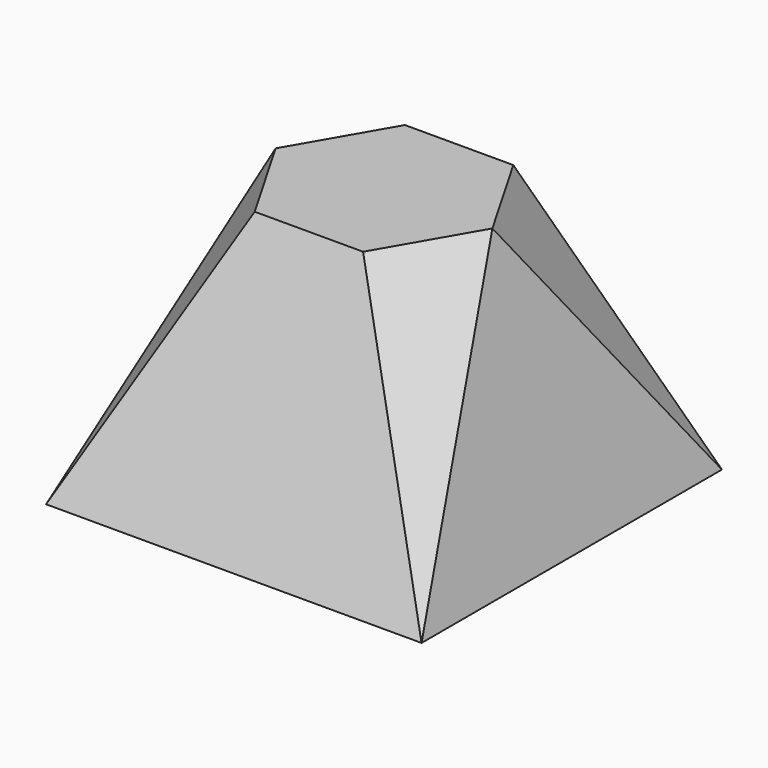
from build123d import *

# Parameters (mm, degrees)
F0_W = 100
F0_H = 100
F3_W = 57.735026919
F3_H = 50


# Not quite as in the source:
# - a feature of the source that left no trace in its solid (it failed there, or was rolled back) is left out
# - a pattern or mirror of a feature is missing from the dataset's text; its kind, count and spacing are read off the source's solid


with BuildPart() as f4:
    # F0 (on Top) → F4 section 0
    with BuildSketch(Plane.XY):
        Rectangle(F0_W, F0_H)
    # F3 (on offset) → F4 section 1
    with BuildSketch(Plane.XY.offset(70)):
        Rectangle(F3_W, F3_H)
    loft()

    # F2 (on offset) → F6 section 0
    with BuildSketch(Plane.XY.offset(70), mode=Mode.PRIVATE) as f6_s0:
        Polygon((28.8675134595, -25), (28.8675134595, 0), (14.4337567297, -25), align=None)
    f6 = loft([f6_s0.sketch, Vertex(50, -50, 0)], mode=Mode.SUBTRACT)

    # F6_copies: F6 across plane
    add(f6.mirror(Plane(origin=(0, 0, 0), x_dir=(0, 0, -1), z_dir=(-1, 0, 0))), mode=Mode.SUBTRACT)

    # F2 (on offset) → F7 section 0
    with BuildSketch(Plane.XY.offset(70), mode=Mode.PRIVATE) as f7_s0:
        Polygon((28.8675134595, 25), (14.4337567297, 25), (28.8675134595, 0), align=None)
    loft([f7_s0.sketch, Vertex(50, 50, 0)], mode=Mode.SUBTRACT)

    # F2 (on offset) → F8 section 0
    with BuildSketch(Plane.XY.offset(70), mode=Mode.PRIVATE) as f8_s0:
        Polygon((-28.8675134595, 0), (-14.4337567297, 25), (-28.8675134595, 25), align=None)
    loft([f8_s0.sketch, Vertex(-50, 50, 0)], mode=Mode.SUBTRACT)


solid = f4.part
